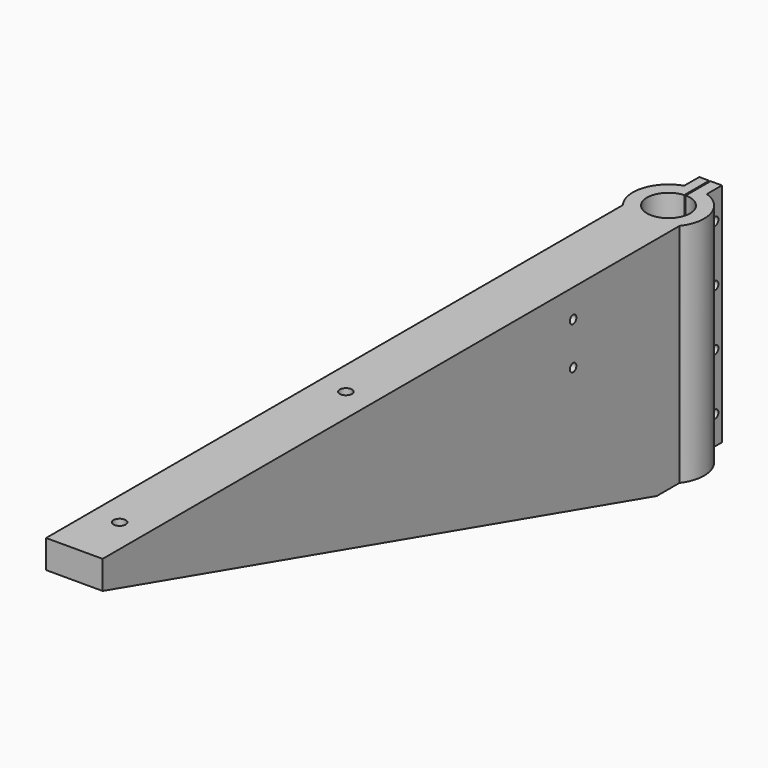
from build123d import *

# Parameters (mm, degrees)
F1_DEPTH  = 80
F0_R      = 7.6
F2_DEPTH  = 80
F3_R      = 2.15
F4_DEPTH  = 80.001
F5_R      = 3.65
F5_R_2    = 2.15
F6_DEPTH  = 70
F8_DEPTH  = 22.601
F10_DEPTH = 80.001
F11_R     = 1.45
F12_DEPTH = 16.601
F13_R     = 1.45
F14_DEPTH = 22.601


with BuildPart() as f1:
    # F0 (on Top) → F1 (new body)
    with BuildSketch(Plane.XY):
        with BuildLine():
            ThreePointArc((10, -7.6655071587), (0, -12.6), (-10, -7.6655071587))
            Line((-10, -7.6655071587), (-10, -262.6))
            Line((-10, -262.6), (10, -262.6))
            Line((10, -262.6), (10, -7.6655071587))
        make_face()
    extrude(amount=-F1_DEPTH)

    # F0 (on Top) → F2 (join)
    with BuildSketch(Plane.XY):
        with BuildLine():
            Line((-4, 18.6), (-4, 11.948221625))
            ThreePointArc((-4, 11.948221625), (-12.0488418199, 3.685839226), (-10, -7.6655071587))
            ThreePointArc((-10, -7.6655071587), (0, -12.6), (10, -7.6655071587))
            ThreePointArc((10, -7.6655071587), (12.0488418199, 3.685839226), (4, 11.948221625))
            Line((4, 11.948221625), (4, 18.6))
            Line((4, 18.6), (-4, 18.6))
        make_face()
        Circle(F0_R, mode=Mode.SUBTRACT)
    extrude(amount=-F2_DEPTH)

    # F3 (on face) → F4 (cut, through all)
    with BuildSketch(Plane.XY):
        with Locations((0, -142.6)):
            Circle(F3_R)
        with Locations((0, -242.6)):
            Circle(F3_R)
    extrude(amount=-F4_DEPTH, mode=Mode.SUBTRACT)

    # F5 (on face) → F6 (cut)
    with BuildSketch(Plane(origin=(0, 0, -80), x_dir=(1, 0, 0), z_dir=(0, 0, -1))):
        with Locations((0, 242.6)):
            Circle(F5_R)
        with Locations((0, 242.6)):
            Circle(F5_R_2, mode=Mode.SUBTRACT)
        with Locations((0, 142.6)):
            Circle(F5_R)
        with Locations((0, 142.6)):
            Circle(F5_R_2, mode=Mode.SUBTRACT)
    extrude(amount=-F6_DEPTH, mode=Mode.SUBTRACT)

    # F7 (on face) → F8 (cut, through all)
    with BuildSketch(Plane.YZ.offset(10)):
        Polygon((-262.6, -80), (-17.6655071587, -80), (-262.6, -10), align=None)
    extrude(amount=-F8_DEPTH, mode=Mode.SUBTRACT)

    # F9 (on face) → F10 (cut, through all)
    with BuildSketch(Plane.XY):
        with BuildLine():
            Line((0, 7.6), (0, 18.6))
            Line((0, 18.6), (-0.5, 18.6))
            Line((-0.5, 18.6), (-0.5, 7.5835347959))
            ThreePointArc((-0.5, 7.5835347959), (-0.2501355147, 7.5958825836), (0, 7.6))
        make_face()
        with BuildLine():
            ThreePointArc((0.5, 7.5835347959), (0.2501355147, 7.5958825836), (0, 7.6))
            Line((0, 7.6), (0, 0))
            Line((0, 0), (0.5, 0))
            Line((0.5, 0), (0.5, 7.5835347959))
        make_face()
        with BuildLine():
            Line((0, 0), (0, 7.6))
            ThreePointArc((0, 7.6), (-0.2501355147, 7.5958825836), (-0.5, 7.5835347959))
            Line((-0.5, 7.5835347959), (-0.5, 0))
            Line((-0.5, 0), (0, 0))
        make_face()
    extrude(amount=-F10_DEPTH, mode=Mode.SUBTRACT)

    # F11 (on face) → F12 (cut, through all)
    with BuildSketch(Plane.YZ.offset(4)):
        with Locations((15.6, -30)):
            Circle(F11_R)
        with Locations((15.6, -70)):
            Circle(F11_R)
        with Locations((15.6, -50)):
            Circle(F11_R)
        with Locations((15.6, -10)):
            Circle(F11_R)
    extrude(amount=-F12_DEPTH, mode=Mode.SUBTRACT)

    # F13 (on face) → F14 (cut, through all)
    with BuildSketch(Plane.YZ.offset(10)):
        with Locations((-54.6655071587, -10)):
            Circle(F13_R)
        with Locations((-54.6655071587, -25)):
            Circle(F13_R)
    extrude(amount=-F14_DEPTH, mode=Mode.SUBTRACT)


solid = f1.part
